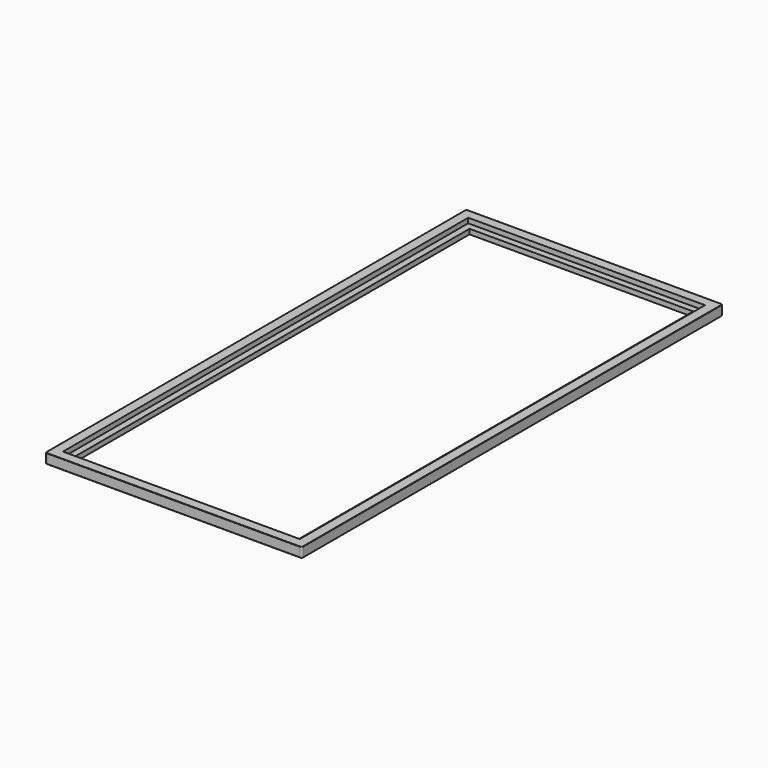
from build123d import *

# Parameters (mm, degrees)
F2_DEPTH     = 19.05
F4_DEPTH     = 19.05
F5_R         = 1.5875
F6_T3_ANGLE  = 90
F6_T6_ANGLE  = 90
F6_T9_ANGLE  = 90
F6_T12_ANGLE = 90
F6_T15_ANGLE = 90
F6_T18_ANGLE = 90
F6_T21_ANGLE = 90
F6_T24_ANGLE = 90
F6_T27_DEPTH = 38.1
F6_T30_DEPTH = 38.1
F6_T33_DEPTH = 38.1
F6_T36_DEPTH = 38.1


# Not quite as in the source:
# - a fillet or chamfer that OpenCascade refuses, or shapes differently, is made with other operations: its cross-section is extruded or revolved along the edge and cut away or added


with BuildPart() as f2:
    # F1 (on Top) → F2 (new body)
    with BuildSketch(Plane.XY):
        Polygon((495.3, -1016), (495.3, 1016), (431.8, 952.5), (431.8, -952.5), align=None)
        Polygon((-431.8, 1016), (-495.3, 1016), (-431.8, 952.5), (431.8, 952.5), (495.3, 1016), align=None)
        Polygon((-431.8, 952.5), (-495.3, 1016), (-495.3, -1016), (-431.8, -952.5), align=None)
        Polygon((-431.8, -952.5), (-495.3, -1016), (431.8, -1016), (495.3, -1016), (431.8, -952.5), align=None)
    extrude(amount=F2_DEPTH)

    # F3 (on face) → F4 (join)
    with BuildSketch(Plane.XY.offset(19.05)):
        Polygon((457.2, -977.9), (-457.2, -977.9), (-495.3, -1016), (495.3, -1016), align=None)
        Polygon((-495.3, -1016), (-457.2, -977.9), (-457.2, 977.9), (-495.3, 1016), align=None)
        Polygon((457.2, 977.9), (457.2, -977.9), (495.3, -1016), (495.3, 1016), align=None)
        Polygon((-495.3, 1016), (-457.2, 977.9), (457.2, 977.9), (495.3, 1016), align=None)
    extrude(amount=F4_DEPTH)

    # F5
    f5_edges = [f2.edges().sort_by_distance(p)[0] for p in [
        (-495.3, 0, 0),
        (-495.3, 0, 38.1),
        (0, -1016, 38.1),
        (0, -1016, 0),
        (495.3, 0, 38.1),
        (495.3, 0, 0),
        (0, 1016, 38.1),
        (0, 1016, 0),
    ]]
    fillet(f5_edges, radius=F5_R)

    # F6: fillet of radius 6.35 on 4 edges, made by hand


with BuildPart() as f6_tool1:
    # F6_s2 → F6_t3 (revolve)
    with BuildSketch(Plane.YZ.offset(488.949034)):
        with BuildLine():
            ThreePointArc((1014.4129, 0), (1015.535432, 0.464968), (1016.0004, 1.5875))
            Line((1016.0004, 1.5875), (1016.0004, 0))
            Line((1016.0004, 0), (1014.4129, 0))
        make_face()
    revolve(axis=Axis((488.949034, 1009.649034, 0), (0, 0, -1)), revolution_arc=F6_T3_ANGLE)


with BuildPart() as f6_tool4:
    # F6_s5 → F6_t6 (revolve)
    with BuildSketch(Plane.XZ.offset(-1009.649034)):
        with BuildLine():
            ThreePointArc((493.7129, 38.1), (494.835432, 37.635032), (495.3004, 36.5125))
            Line((495.3004, 36.5125), (495.3004, 38.1))
            Line((495.3004, 38.1), (493.7129, 38.1))
        make_face()
    revolve(axis=Axis((488.949034, 1009.649034, 38.1), (0, 0, 1)), revolution_arc=F6_T6_ANGLE)


with BuildPart() as f6_tool7:
    # F6_s8 → F6_t9 (revolve)
    with BuildSketch(Plane.YZ.offset(488.949034)):
        with BuildLine():
            ThreePointArc((-1014.4129, 38.1), (-1015.535432, 37.635032), (-1016.0004, 36.5125))
            Line((-1016.0004, 36.5125), (-1016.0004, 38.1))
            Line((-1016.0004, 38.1), (-1014.4129, 38.1))
        make_face()
    revolve(axis=Axis((488.949034, -1009.649034, 38.1), (0, 0, 1)), revolution_arc=F6_T9_ANGLE)


with BuildPart() as f6_tool10:
    # F6_s11 → F6_t12 (revolve)
    with BuildSketch(Plane.XZ.offset(1009.649034)):
        with BuildLine():
            ThreePointArc((493.7129, 0), (494.835432, 0.464968), (495.3004, 1.5875))
            Line((495.3004, 1.5875), (495.3004, 0))
            Line((495.3004, 0), (493.7129, 0))
        make_face()
    revolve(axis=Axis((488.949034, -1009.649034, 0), (0, 0, -1)), revolution_arc=F6_T12_ANGLE)


with BuildPart() as f6_tool13:
    # F6_s14 → F6_t15 (revolve)
    with BuildSketch(Plane.XZ.offset(1009.649034)):
        with BuildLine():
            ThreePointArc((-493.7129, 38.1), (-494.835432, 37.635032), (-495.3004, 36.5125))
            Line((-495.3004, 36.5125), (-495.3004, 38.1))
            Line((-495.3004, 38.1), (-493.7129, 38.1))
        make_face()
    revolve(axis=Axis((-488.949034, -1009.649034, 38.1), (0, 0, 1)), revolution_arc=F6_T15_ANGLE)


with BuildPart() as f6_tool16:
    # F6_s17 → F6_t18 (revolve)
    with BuildSketch(Plane.YZ.offset(-488.949034)):
        with BuildLine():
            ThreePointArc((-1014.4129, 0), (-1015.535432, 0.464968), (-1016.0004, 1.5875))
            Line((-1016.0004, 1.5875), (-1016.0004, 0))
            Line((-1016.0004, 0), (-1014.4129, 0))
        make_face()
    revolve(axis=Axis((-488.949034, -1009.649034, 0), (0, 0, -1)), revolution_arc=F6_T18_ANGLE)


with BuildPart() as f6_tool19:
    # F6_s20 → F6_t21 (revolve)
    with BuildSketch(Plane.XZ.offset(-1009.649034)):
        with BuildLine():
            ThreePointArc((-493.7129, 0), (-494.835432, 0.464968), (-495.3004, 1.5875))
            Line((-495.3004, 1.5875), (-495.3004, 0))
            Line((-495.3004, 0), (-493.7129, 0))
        make_face()
    revolve(axis=Axis((-488.949034, 1009.649034, 0), (0, 0, -1)), revolution_arc=F6_T21_ANGLE)


with BuildPart() as f6_tool22:
    # F6_s23 → F6_t24 (revolve)
    with BuildSketch(Plane.YZ.offset(-488.949034)):
        with BuildLine():
            ThreePointArc((1014.4129, 38.1), (1015.535432, 37.635032), (1016.0004, 36.5125))
            Line((1016.0004, 36.5125), (1016.0004, 38.1))
            Line((1016.0004, 38.1), (1014.4129, 38.1))
        make_face()
    revolve(axis=Axis((-488.949034, 1009.649034, 38.1), (0, 0, 1)), revolution_arc=F6_T24_ANGLE)


with BuildPart() as f6_tool25:
    # F6_s26 → F6_t27 (new body)
    with BuildSketch(Plane.XY):
        with BuildLine():
            ThreePointArc((-488.949034, 1016.0004), (-493.440128, 1014.140128), (-495.3004, 1009.649034))
            Line((-495.3004, 1009.649034), (-495.935537, 1009.649034))
            ThreePointArc((-495.935537, 1009.649034), (-495.935137, 1012.824517), (-495.935137, 1016))
            Line((-495.935137, 1016), (-495.3, 1016.635137))
            ThreePointArc((-495.3, 1016.635137), (-492.124517, 1016.635137), (-488.949034, 1016.635537))
            Line((-488.949034, 1016.635537), (-488.949034, 1016.0004))
        make_face()
    extrude(amount=F6_T27_DEPTH)


with BuildPart() as f6_tool28:
    # F6_s29 → F6_t30 (new body)
    with BuildSketch(Plane.XY.offset(38.1)):
        with BuildLine():
            ThreePointArc((-488.949034, -1016.0004), (-493.440128, -1014.140128), (-495.3004, -1009.649034))
            Line((-495.3004, -1009.649034), (-495.935537, -1009.649034))
            ThreePointArc((-495.935537, -1009.649034), (-495.935137, -1012.824517), (-495.935137, -1016))
            Line((-495.935137, -1016), (-495.3, -1016.635137))
            ThreePointArc((-495.3, -1016.635137), (-492.124517, -1016.635137), (-488.949034, -1016.635537))
            Line((-488.949034, -1016.635537), (-488.949034, -1016.0004))
        make_face()
    extrude(amount=-F6_T30_DEPTH)


with BuildPart() as f6_tool31:
    # F6_s32 → F6_t33 (new body)
    with BuildSketch(Plane.XY.offset(38.1)):
        with BuildLine():
            ThreePointArc((495.3004, -1009.649034), (493.440128, -1014.140128), (488.949034, -1016.0004))
            Line((488.949034, -1016.0004), (488.949034, -1016.635537))
            ThreePointArc((488.949034, -1016.635537), (492.124517, -1016.635137), (495.3, -1016.635137))
            Line((495.3, -1016.635137), (495.935137, -1016))
            ThreePointArc((495.935137, -1016), (495.935137, -1012.824517), (495.935537, -1009.649034))
            Line((495.935537, -1009.649034), (495.3004, -1009.649034))
        make_face()
    extrude(amount=-F6_T33_DEPTH)


with BuildPart() as f6_tool34:
    # F6_s35 → F6_t36 (new body)
    with BuildSketch(Plane.XY):
        with BuildLine():
            ThreePointArc((495.3004, 1009.649034), (493.440128, 1014.140128), (488.949034, 1016.0004))
            Line((488.949034, 1016.0004), (488.949034, 1016.635537))
            ThreePointArc((488.949034, 1016.635537), (492.124517, 1016.635137), (495.3, 1016.635137))
            Line((495.3, 1016.635137), (495.935137, 1016))
            ThreePointArc((495.935137, 1016), (495.935137, 1012.824517), (495.935537, 1009.649034))
            Line((495.935537, 1009.649034), (495.3004, 1009.649034))
        make_face()
    extrude(amount=F6_T36_DEPTH)


with BuildPart() as f2_1:
    add(f2.part)

    # F6_t37: cut F6_tool1, F6_tool4, F6_tool7, F6_tool10, F6_tool13, F6_tool16, F6_tool19, F6_tool22, F6_tool25, F6_tool28, F6_tool31, F6_tool34
    add([f6_tool1.part, f6_tool4.part, f6_tool7.part, f6_tool10.part, f6_tool13.part, f6_tool16.part, f6_tool19.part, f6_tool22.part, f6_tool25.part, f6_tool28.part, f6_tool31.part, f6_tool34.part], mode=Mode.SUBTRACT)


solid = f2_1.part
